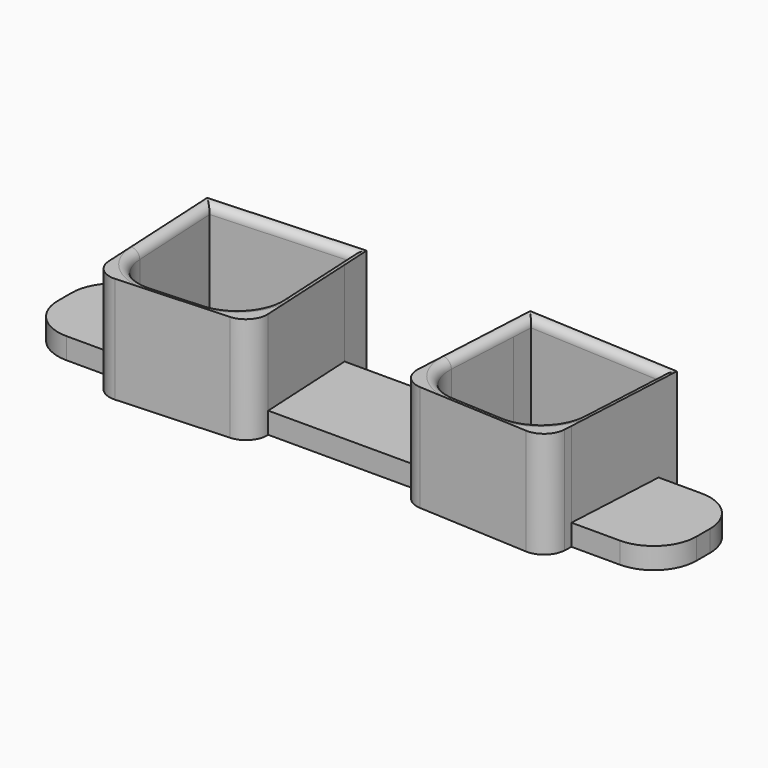
from build123d import *

# Parameters (mm, degrees)
F1_DEPTH     = 25
F2_DEPTH     = 5
F3_R         = 10
F4_R         = 5
F6_T1_DEPTH  = 22
F6_T3_DEPTH  = 32
F6_T5_DEPTH  = 32
F6_T7_DEPTH  = 22
F6_T9_DEPTH  = 22
F6_T11_DEPTH = 12
F6_T13_DEPTH = 22
F6_T15_DEPTH = 12
F6_T18_ANGLE = 90
F6_T20_ANGLE = 90
F6_T22_ANGLE = 90
F6_T24_ANGLE = 90
F6_T29_DEPTH = 37
F6_T34_DEPTH = 27
F6_T42_DEPTH = 37
F6_T47_DEPTH = 27
F6_T55_DEPTH = 27
F6_T60_DEPTH = 37
F6_T68_DEPTH = 27
F6_T73_DEPTH = 37


# Not quite as in the source:
# - a fillet or chamfer that OpenCascade refuses, or shapes differently, is made with other operations: its cross-section is extruded or revolved along the edge and cut away or added
# - a feature names something its author has since deleted; it is built from what else it names


with BuildPart() as f1:
    # F0 (on Top) → F1 (new body)
    with BuildSketch(Plane.XY):
        Polygon((-52.9008508874, 12), (-53.065447856, 15.1406972562), (-21.1093027438, 16.815447856), (-20.8569358154, 12), (-18.8541911234, 12), (-19.2167155868, 18.917378838), (-55.167378838, 17.0332844132), (-54.9035955794, 12), align=None)
        Polygon((-51.6430641846, -12), (-52.9008508874, 12), (-54.9035955794, 12), (-53.6458088766, -12), align=None)
        Polygon((-18.8541911234, 12), (-20.8569358154, 12), (-19.5991491126, -12), (-17.5964044206, -12), align=None)
        Polygon((-51.3906972562, -16.815447856), (-51.6430641846, -12), (-53.6458088766, -12), (-53.2832844132, -18.917378838), (-17.332621162, -17.0332844132), (-17.5964044206, -12), (-19.5991491126, -12), (-19.434552144, -15.1406972562), align=None)
    extrude(amount=F1_DEPTH)

    # F0 (on Top) → F2 (join)
    with BuildSketch(Plane.XY):
        Polygon((-53.6458088766, -12), (-54.9035955794, 12), (-75, 12), (-75, -12), align=None)
        Polygon((0, 12), (-18.8541911234, 12), (-17.5964044206, -12), (0, -12), align=None)
    extrude(amount=F2_DEPTH)

    # F3
    f3_edges = [f1.edges().sort_by_distance(p)[0] for p in [
        (-75, -12, 2.5),
        (-75, 12, 2.5),
        (-51.390697, -16.815448, 12.5),
        (-19.434552, -15.140697, 12.5),
    ]]
    fillet(f3_edges, radius=F3_R)

    # F4
    f4_edges = [f1.edges().sort_by_distance(p)[0] for p in [
        (-53.283284, -18.917379, 12.5),
        (-17.332621, -17.033284, 12.5),
    ]]
    fillet(f4_edges, radius=F4_R)

    # F5: F1 across plane


with BuildPart() as f1_1:
    add(f1.part)
    add(f1.part.mirror(Plane.YZ))

    # F6: fillet of radius 2 on 12 edges, made by hand

    # F6_s2 → F6_t1 (cut)
    with BuildSketch(Plane(origin=(0.214725091, -4.0971988118, 0), x_dir=(0, 0, 1), z_dir=(-0.0523359562, 0.9986295348, 0))):
        with BuildLine():
            ThreePointArc((25, -54.2003206349), (24.4142135624, -52.7861070725), (23, -52.2003206349))
            Line((23, -52.2003206349), (25, -52.2003206349))
            Line((25, -52.2003206349), (25, -54.2003206349))
        make_face()
    extrude(amount=F6_T1_DEPTH, mode=Mode.SUBTRACT)

    # F6_s4 → F6_t3 (cut)
    with BuildSketch(Plane(origin=(-52.1287819096, -2.7319536966, 0), x_dir=(0, 0, 1), z_dir=(0.9986295348, 0.0523359562, 0))):
        with BuildLine():
            ThreePointArc((23, -17.8971784138), (24.4142135624, -18.4829648514), (25, -19.8971784138))
            Line((25, -19.8971784138), (25, -17.8971784138))
            Line((25, -17.8971784138), (23, -17.8971784138))
        make_face()
    extrude(amount=F6_T3_DEPTH, mode=Mode.SUBTRACT)

    # F6_s6 → F6_t5 (cut)
    with BuildSketch(Plane(origin=(52.1287819096, -2.7319536966, 0), x_dir=(0, 0, 1), z_dir=(-0.9986295348, 0.0523359562, 0))):
        with BuildLine():
            ThreePointArc((25, 19.8971784138), (24.4142135624, 18.4829648514), (23, 17.8971784138))
            Line((23, 17.8971784138), (25, 17.8971784138))
            Line((25, 17.8971784138), (25, 19.8971784138))
        make_face()
    extrude(amount=F6_T5_DEPTH, mode=Mode.SUBTRACT)

    # F6_s8 → F6_t7 (cut)
    with BuildSketch(Plane(origin=(-0.214725091, -4.0971988118, 0), x_dir=(0, 0, 1), z_dir=(0.0523359562, 0.9986295348, 0))):
        with BuildLine():
            ThreePointArc((23, 52.2003206349), (24.4142135624, 52.7861070725), (25, 54.2003206349))
            Line((25, 54.2003206349), (25, 52.2003206349))
            Line((25, 52.2003206349), (23, 52.2003206349))
        make_face()
    extrude(amount=F6_T7_DEPTH, mode=Mode.SUBTRACT)

    # F6_s10 → F6_t9 (cut)
    with BuildSketch(Plane(origin=(0.9366659463, 17.8726509528, 0), x_dir=(0, 0, 1), z_dir=(-0.0523359562, -0.9986295348, 0))):
        with BuildLine():
            ThreePointArc((25, -18.2003206349), (24.4142135624, -19.6145341972), (23, -20.2003206349))
            Line((23, -20.2003206349), (25, -20.2003206349))
            Line((25, -20.2003206349), (25, -18.2003206349))
        make_face()
    extrude(amount=F6_T9_DEPTH, mode=Mode.SUBTRACT)

    # F6_s12 → F6_t11 (cut)
    with BuildSketch(Plane(origin=(30.158932145, -1.5805626593, 0), x_dir=(0, 0, 1), z_dir=(0.9986295348, -0.0523359562, 0))):
        with BuildLine():
            ThreePointArc((25, 16.1028215862), (24.4142135624, 14.6886080238), (23, 14.1028215862))
            Line((23, 14.1028215862), (25, 14.1028215862))
            Line((25, 14.1028215862), (25, 16.1028215862))
        make_face()
    extrude(amount=F6_T11_DEPTH, mode=Mode.SUBTRACT)

    # F6_s14 → F6_t13 (cut)
    with BuildSketch(Plane(origin=(-0.9366659463, 17.8726509528, 0), x_dir=(0, 0, 1), z_dir=(0.0523359562, -0.9986295348, 0))):
        with BuildLine():
            ThreePointArc((25, 18.2003206349), (24.4142135624, 19.6145341972), (23, 20.2003206349))
            Line((23, 20.2003206349), (25, 20.2003206349))
            Line((25, 20.2003206349), (25, 18.2003206349))
        make_face()
    extrude(amount=F6_T13_DEPTH, mode=Mode.SUBTRACT)

    # F6_s16 → F6_t15 (cut)
    with BuildSketch(Plane(origin=(-30.158932145, -1.5805626593, 0), x_dir=(0, 0, 1), z_dir=(-0.9986295348, -0.0523359562, 0))):
        with BuildLine():
            ThreePointArc((25, -16.1028215862), (24.4142135624, -14.6886080238), (23, -14.1028215862))
            Line((23, -14.1028215862), (25, -14.1028215862))
            Line((25, -14.1028215862), (25, -16.1028215862))
        make_face()
    extrude(amount=F6_T15_DEPTH, mode=Mode.SUBTRACT)

    # F6_s17 → F6_t18 (revolve, cut)
    with BuildSketch(Plane(origin=(-42.1424865621, -2.2085941342, 0), x_dir=(0, 0, 1), z_dir=(0.9986295348, 0.0523359562, 0))):
        with BuildLine():
            ThreePointArc((25, 16.1028215862), (24.4142135624, 14.6886080238), (23, 14.1028215862))
            Line((23, 14.1028215862), (25, 14.1028215862))
            Line((25, 14.1028215862), (25, 16.1028215862))
        make_face()
    revolve(axis=Axis((-41.9277614711, -6.305792946, 25), (0, 0, -1)), revolution_arc=F6_T18_ANGLE, mode=Mode.SUBTRACT)

    # F6_s19 → F6_t20 (revolve, cut)
    with BuildSketch(Plane(origin=(-0.214725091, -4.0971988118, 0), x_dir=(0, 0, 1), z_dir=(0.0523359562, 0.9986295348, 0))):
        with BuildLine():
            ThreePointArc((25, 18.2003206349), (24.4142135624, 19.6145341972), (23, 20.2003206349))
            Line((23, 20.2003206349), (25, 20.2003206349))
            Line((25, 20.2003206349), (25, 18.2003206349))
        make_face()
    revolve(axis=Axis((29.944207054, -5.6777614711, 25), (0, 0, 1)), revolution_arc=F6_T20_ANGLE, mode=Mode.SUBTRACT)

    # F6_s21 → F6_t22 (revolve, cut)
    with BuildSketch(Plane(origin=(42.1424865621, -2.2085941342, 0), x_dir=(0, 0, 1), z_dir=(-0.9986295348, 0.0523359562, 0))):
        with BuildLine():
            ThreePointArc((25, -16.1028215862), (24.4142135624, -14.6886080238), (23, -14.1028215862))
            Line((23, -14.1028215862), (25, -14.1028215862))
            Line((25, -14.1028215862), (25, -16.1028215862))
        make_face()
    revolve(axis=Axis((41.9277614711, -6.305792946, 25), (0, 0, 1)), revolution_arc=F6_T22_ANGLE, mode=Mode.SUBTRACT)

    # F6_s23 → F6_t24 (revolve, cut)
    with BuildSketch(Plane(origin=(0.214725091, -4.0971988118, 0), x_dir=(0, 0, 1), z_dir=(-0.0523359562, 0.9986295348, 0))):
        with BuildLine():
            ThreePointArc((25, -18.2003206349), (24.4142135624, -19.6145341972), (23, -20.2003206349))
            Line((23, -20.2003206349), (25, -20.2003206349))
            Line((25, -20.2003206349), (25, -18.2003206349))
        make_face()
    revolve(axis=Axis((-29.944207054, -5.6777614711, 25), (0, 0, -1)), revolution_arc=F6_T24_ANGLE, mode=Mode.SUBTRACT)


with BuildPart() as f6_tool27:
    # F6_s28 → F6_t29 (new body)
    with BuildSketch(Plane(origin=(-57.1219295834, -2.9936334778, 0), x_dir=(0, 0, 1), z_dir=(0.9986295348, 0.0523359562, 0))):
        with BuildLine():
            ThreePointArc((23, -17.8971784138), (24.4142135624, -18.4829648514), (25, -19.8971784138))
            Line((25, -19.8971784138), (25, -17.8971784138))
            Line((25, -17.8971784138), (23, -17.8971784138))
        make_face()
    extrude(amount=F6_T29_DEPTH)

    split(bisect_by=Plane(origin=(-52.1287819096, -2.7319536966, 0), x_dir=(0, 0, 1), z_dir=(-0.9986295348, -0.0523359562, 0)), keep=Keep.TOP)

    split(bisect_by=Plane(origin=(-54.1260409791, -2.8366256091, 0), x_dir=(0, 0, 1), z_dir=(0.9986295348, 0.0523359562, 0)), keep=Keep.TOP)


with BuildPart() as f6_tool32:
    # F6_s33 → F6_t34 (new body)
    with BuildSketch(Plane(origin=(0.214725091, -4.0971988118, 0), x_dir=(0, 0, 1), z_dir=(-0.0523359562, 0.9986295348, 0))):
        with BuildLine():
            ThreePointArc((25, -54.2003206349), (24.4142135624, -52.7861070725), (23, -52.2003206349))
            Line((23, -52.2003206349), (25, -52.2003206349))
            Line((25, -52.2003206349), (25, -54.2003206349))
        make_face()
    extrude(amount=F6_T34_DEPTH)

    split(bisect_by=Plane(origin=(-0.9366659463, 17.8726509528, 0), x_dir=(0, 0, 1), z_dir=(-0.0523359562, 0.9986295348, 0)), keep=Keep.TOP)

    split(bisect_by=Plane(origin=(-1.0413378588, 19.8699100223, 0), x_dir=(0, 0, 1), z_dir=(0.0523359562, -0.9986295348, 0)), keep=Keep.TOP)


with BuildPart() as f6_tool27_1:
    add(f6_tool27.part)

    # F6_t37: intersect F6_tool32
    add(f6_tool32.part, mode=Mode.INTERSECT)


with BuildPart() as f1_2:
    add(f1_1.part)

    # F6_t25: cut F6_tool27
    add(f6_tool27_1.part, mode=Mode.SUBTRACT)


with BuildPart() as f6_tool40:
    # F6_s41 → F6_t42 (new body)
    with BuildSketch(Plane(origin=(-52.1287819096, -2.7319536966, 0), x_dir=(0, 0, 1), z_dir=(0.9986295348, 0.0523359562, 0))):
        with BuildLine():
            ThreePointArc((23, -17.8971784138), (24.4142135624, -18.4829648514), (25, -19.8971784138))
            Line((25, -19.8971784138), (25, -17.8971784138))
            Line((25, -17.8971784138), (23, -17.8971784138))
        make_face()
    extrude(amount=F6_T42_DEPTH)

    split(bisect_by=Plane(origin=(-20.1726367975, -1.0572030968, 0), x_dir=(0, 0, 1), z_dir=(0.9986295348, 0.0523359562, 0)), keep=Keep.TOP)

    split(bisect_by=Plane(origin=(-18.175377728, -0.9525311844, 0), x_dir=(0, 0, 1), z_dir=(-0.9986295348, -0.0523359562, 0)), keep=Keep.TOP)


with BuildPart() as f6_tool45:
    # F6_s46 → F6_t47 (new body)
    with BuildSketch(Plane(origin=(-1.1983457276, 22.8657986266, 0), x_dir=(0, 0, 1), z_dir=(0.0523359562, -0.9986295348, 0))):
        with BuildLine():
            ThreePointArc((25, 18.2003206349), (24.4142135624, 19.6145341972), (23, 20.2003206349))
            Line((23, 20.2003206349), (25, 20.2003206349))
            Line((25, 20.2003206349), (25, 18.2003206349))
        make_face()
    extrude(amount=F6_T47_DEPTH)

    split(bisect_by=Plane(origin=(-0.9366659463, 17.8726509528, 0), x_dir=(0, 0, 1), z_dir=(-0.0523359562, 0.9986295348, 0)), keep=Keep.TOP)

    split(bisect_by=Plane(origin=(-1.0413378588, 19.8699100223, 0), x_dir=(0, 0, 1), z_dir=(0.0523359562, -0.9986295348, 0)), keep=Keep.TOP)


with BuildPart() as f6_tool40_1:
    add(f6_tool40.part)

    # F6_t50: intersect F6_tool45
    add(f6_tool45.part, mode=Mode.INTERSECT)


with BuildPart() as f1_3:
    add(f1_2.part)

    # F6_t38: cut F6_tool40
    add(f6_tool40_1.part, mode=Mode.SUBTRACT)


with BuildPart() as f6_tool53:
    # F6_s54 → F6_t55 (new body)
    with BuildSketch(Plane(origin=(-0.214725091, -4.0971988118, 0), x_dir=(0, 0, 1), z_dir=(0.0523359562, 0.9986295348, 0))):
        with BuildLine():
            ThreePointArc((23, 52.2003206349), (24.4142135624, 52.7861070725), (25, 54.2003206349))
            Line((25, 54.2003206349), (25, 52.2003206349))
            Line((25, 52.2003206349), (23, 52.2003206349))
        make_face()
    extrude(amount=F6_T55_DEPTH)

    split(bisect_by=Plane(origin=(0.9366659463, 17.8726509528, 0), x_dir=(0, 0, 1), z_dir=(0.0523359562, 0.9986295348, 0)), keep=Keep.TOP)

    split(bisect_by=Plane(origin=(1.0413378588, 19.8699100223, 0), x_dir=(0, 0, 1), z_dir=(-0.0523359562, -0.9986295348, 0)), keep=Keep.TOP)


with BuildPart() as f6_tool58:
    # F6_s59 → F6_t60 (new body)
    with BuildSketch(Plane(origin=(57.1219295834, -2.9936334778, 0), x_dir=(0, 0, 1), z_dir=(-0.9986295348, 0.0523359562, 0))):
        with BuildLine():
            ThreePointArc((25, 19.8971784138), (24.4142135624, 18.4829648514), (23, 17.8971784138))
            Line((23, 17.8971784138), (25, 17.8971784138))
            Line((25, 17.8971784138), (25, 19.8971784138))
        make_face()
    extrude(amount=F6_T60_DEPTH)

    split(bisect_by=Plane(origin=(52.1287819096, -2.7319536966, 0), x_dir=(0, 0, 1), z_dir=(0.9986295348, -0.0523359562, 0)), keep=Keep.TOP)

    split(bisect_by=Plane(origin=(54.1260409791, -2.8366256091, 0), x_dir=(0, 0, 1), z_dir=(-0.9986295348, 0.0523359562, 0)), keep=Keep.TOP)


with BuildPart() as f6_tool53_1:
    add(f6_tool53.part)

    # F6_t63: intersect F6_tool58
    add(f6_tool58.part, mode=Mode.INTERSECT)


with BuildPart() as f1_4:
    add(f1_3.part)

    # F6_t51: cut F6_tool53
    add(f6_tool53_1.part, mode=Mode.SUBTRACT)


with BuildPart() as f6_tool66:
    # F6_s67 → F6_t68 (new body)
    with BuildSketch(Plane(origin=(1.1983457276, 22.8657986266, 0), x_dir=(0, 0, 1), z_dir=(-0.0523359562, -0.9986295348, 0))):
        with BuildLine():
            ThreePointArc((25, -18.2003206349), (24.4142135624, -19.6145341972), (23, -20.2003206349))
            Line((23, -20.2003206349), (25, -20.2003206349))
            Line((25, -20.2003206349), (25, -18.2003206349))
        make_face()
    extrude(amount=F6_T68_DEPTH)

    split(bisect_by=Plane(origin=(0.9366659463, 17.8726509528, 0), x_dir=(0, 0, 1), z_dir=(0.0523359562, 0.9986295348, 0)), keep=Keep.TOP)

    split(bisect_by=Plane(origin=(1.0413378588, 19.8699100223, 0), x_dir=(0, 0, 1), z_dir=(-0.0523359562, -0.9986295348, 0)), keep=Keep.TOP)


with BuildPart() as f6_tool71:
    # F6_s72 → F6_t73 (new body)
    with BuildSketch(Plane(origin=(52.1287819096, -2.7319536966, 0), x_dir=(0, 0, 1), z_dir=(-0.9986295348, 0.0523359562, 0))):
        with BuildLine():
            ThreePointArc((25, 19.8971784138), (24.4142135624, 18.4829648514), (23, 17.8971784138))
            Line((23, 17.8971784138), (25, 17.8971784138))
            Line((25, 17.8971784138), (25, 19.8971784138))
        make_face()
    extrude(amount=F6_T73_DEPTH)

    split(bisect_by=Plane(origin=(20.1726367975, -1.0572030968, 0), x_dir=(0, 0, 1), z_dir=(-0.9986295348, 0.0523359562, 0)), keep=Keep.TOP)

    split(bisect_by=Plane(origin=(18.175377728, -0.9525311844, 0), x_dir=(0, 0, 1), z_dir=(0.9986295348, -0.0523359562, 0)), keep=Keep.TOP)


with BuildPart() as f6_tool66_1:
    add(f6_tool66.part)

    # F6_t76: intersect F6_tool71
    add(f6_tool71.part, mode=Mode.INTERSECT)


with BuildPart() as f1_5:
    add(f1_4.part)

    # F6_t64: cut F6_tool66
    add(f6_tool66_1.part, mode=Mode.SUBTRACT)


solid = f1_5.part
